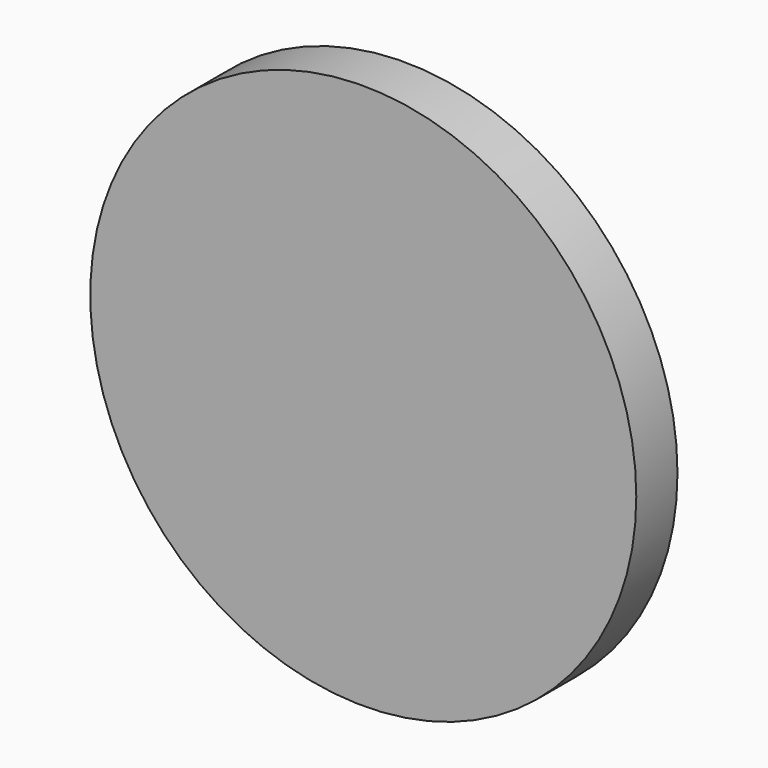
from build123d import *

# Parameters (mm, degrees)
F0_R         = 10.605
F1_DEPTH     = 2
F2_TEXT_SIZE = 17.3793109651
F3_DEPTH     = 0.5


# Not quite as in the source:
# - Text() gives the source's letters only with a copy of the font that has no kerning and outlines rounded to 1/6400 em; it was checked with that copy


with BuildPart() as f1:
    # F0 (on Front) → F1 (new body)
    with BuildSketch(Plane.XZ):
        Circle(F0_R)
    extrude(amount=F1_DEPTH)

    # F2 (on face) → F3 (join)
    with BuildSketch(Plane(origin=(0, 0, 0), x_dir=(-1, 0, 0), z_dir=(0, 1, 0))):
        with Locations((-5.0240908749, -6.2274983502)):
            Text('5', F2_TEXT_SIZE, font='Open Sans', text_align=(TextAlign.LEFT, TextAlign.BOTTOM))
    extrude(amount=F3_DEPTH)


solid = f1.part
